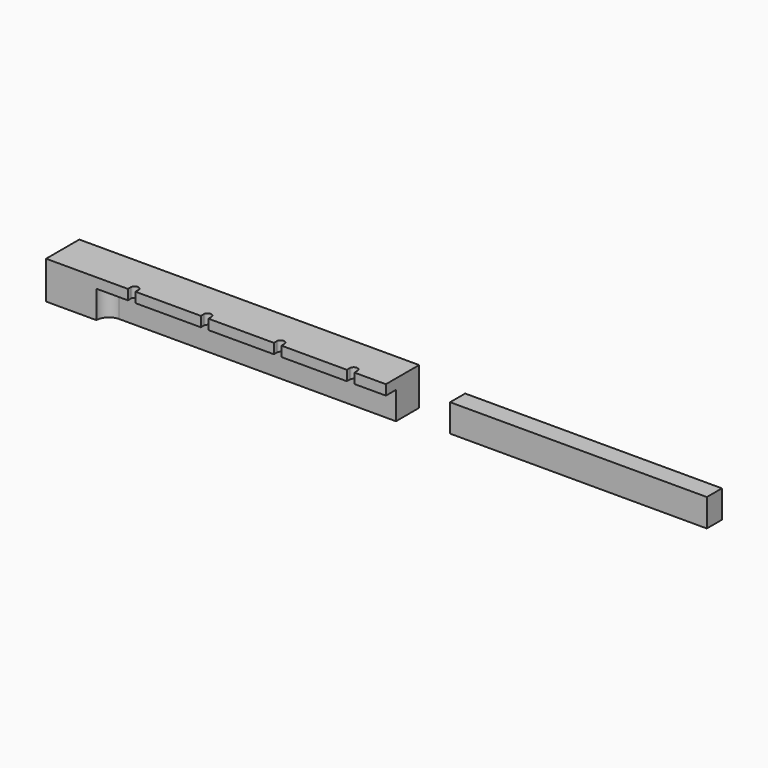
from build123d import *

# Parameters (mm, degrees)
F1_DEPTH = 4
F3_DEPTH = 11
F5_W     = 7.5
F5_H     = 11
F6_DEPTH = 51
F7_R     = 4.99999


# Not quite as in the source:
# - a fillet or chamfer is up to 0.001 mm smaller than in the source, because OpenCascade refuses the exact size


with BuildPart() as f1:
    # F0 (on Top) → F1 (new body)
    with BuildSketch(Plane.XY):
        with BuildLine():
            Line((55, 0), (67.5, 0))
            Line((67.5, 0), (67.5, 16.5))
            Line((67.5, 16.5), (-67.5, 16.5))
            Line((-67.5, 16.5), (-67.5, 0))
            Line((-67.5, 0), (-35, 0))
            Line((-35, 0), (-35, 1.5))
            ThreePointArc((-35, 1.5), (-33.5, 3), (-32, 1.5))
            Line((-32, 1.5), (-32, 0))
            Line((-32, 0), (-6, 0))
            Line((-6, 0), (-6, 1.5))
            ThreePointArc((-6, 1.5), (-4.5, 3), (-3, 1.5))
            Line((-3, 1.5), (-3, 0))
            Line((-3, 0), (23, 0))
            Line((23, 0), (23, 1.5))
            ThreePointArc((23, 1.5), (24.5, 3), (26, 1.5))
            Line((26, 1.5), (26, 0))
            Line((26, 0), (52, 0))
            Line((52, 0), (52, 1.5))
            ThreePointArc((52, 1.5), (53.5, 3), (55, 1.5))
            Line((55, 1.5), (55, 0))
        make_face()
    extrude(amount=F1_DEPTH)

    # F2 (on face) → F3 (join)
    with BuildSketch(Plane(origin=(0, 0, 0), x_dir=(1, 0, 0), z_dir=(0, 0, -1))):
        Polygon((67.5, -16.5), (67.5, -4.9999998882), (-47.5, -4.9999998882), (-47.5, 0), (-67.5, 0), (-67.5, -16.5), align=None)
    extrude(amount=F3_DEPTH)

    # F7 (radius 5 in the source; OpenCascade refuses exactly that, so slightly less here)
    f7_edges = [f1.edges().sort_by_distance(p)[0] for p in [
        (-47.5, 5, -5.5),
    ]]
    fillet(f7_edges, radius=F7_R)


with BuildPart() as f6:
    # F5 (on offset) → F6 (new body, symmetric)
    with BuildSketch(Plane.YZ.offset(150)):
        with Locations((-3.75, 5.5)):
            Rectangle(F5_W, F5_H)
    extrude(amount=F6_DEPTH, both=True)


solid = Compound([f1.part, f6.part])
